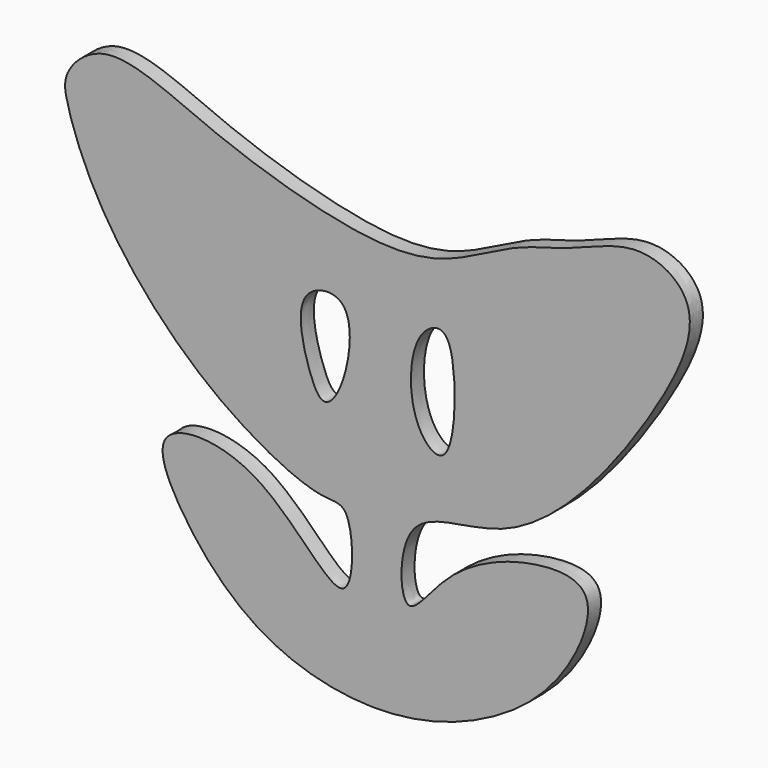
from build123d import *

# Parameters (mm, degrees)
F1_DEPTH = 2
F3_DEPTH = 25


with BuildPart() as f1:
    # F0 (on Front) → F1 (new body)
    with BuildSketch(Plane.XZ):
        with BuildLine():
            add(Edge.make_bspline(
                [(-75.8347990971, 56.2486425042), (-75.1836263652, 57.6802689805), (-70.9340790333, 61.7640658934), (-58.7880150697, 55.6323601286), (-43.4543911865, 50.6624350906), (-30.7629702937, 49.5047020163), (-21.2430871182, 55.7381469131), (-14.4280411182, 56.8600440589), (-5.9908935153, 61.2392779803), (2.5977107271, 56.1596013405), (-3.7766212938, 42.0301545009), (-19.9171824428, 21.4464982023), (-35.5090674399, 24.204165931), (-35.1659184419, 8.7502373537), (-29.3709449572, 18.4771355864), (-19.1906116712, 22.527164785), (-10.2486183797, 21.8239112152), (-14.7448810071, 9.9497124678), (-24.7301847276, 2.2972307162), (-37.8974817036, -1.1632111012), (-52.6991606842, 2.3225134129), (-61.8943580671, 12.4158839786), (-66.5312753548, 22.7161079835), (-51.5232135092, 22.7569790255), (-40.576550772, 5.5851938951), (-40.8518766389, 21.2862833862), (-45.3318688846, 20.0077827884), (-59.5970602772, 27.2946481454), (-71.9458419573, 41.6440588858), (-75.9609853522, 52.4043003525), (-76.3433099111, 55.1306633428), (-75.8347990971, 56.2486425042)],
                knots=[0, 0, 0, 0, 0.0253349266, 0.0628814506, 0.1064129014, 0.1436333956, 0.1780743263, 0.2061872931, 0.2378149533, 0.2655878625, 0.304558889, 0.3583719074, 0.3954019389, 0.4254899915, 0.4524182936, 0.4893046572, 0.5153680757, 0.5480343317, 0.586157669, 0.6246036867, 0.6649227249, 0.7046153879, 0.733595282, 0.7687775312, 0.8078125444, 0.8378755979, 0.8566485225, 0.8978413978, 0.9453852813, 0.9802155657, 1, 1, 1, 1], degree=3))
        make_face()
    extrude(amount=F1_DEPTH)

    # F2 (on face) → F3 (cut)
    with BuildSketch(Plane.XZ.offset(2)):
        with BuildLine():
            add(Edge.make_bspline(
                [(-42.2871634364, 42.2871671617), (-40.7233235578, 40.7460702061), (-41.6404243336, 33.64294769), (-44.5487515397, 29.883684324), (-46.6450188115, 34.0930294047), (-48.5043967712, 42.6275810256), (-43.3972597055, 43.3811193011), (-42.2871634364, 42.2871671617)],
                knots=[0, 0, 0, 0, 0.25425656, 0.4151017388, 0.5773983635, 0.8195152442, 1, 1, 1, 1], degree=3))
        make_face()
        with BuildLine():
            add(Edge.make_bspline(
                [(-32.8900180757, 41.4816960692), (-34.1259395093, 39.117633331), (-34.1810178637, 32.0726846499), (-28.7069781951, 27.6905511122), (-28.1052302328, 39.4105956249), (-29.6890897505, 44.3984102877), (-32.160134876, 42.8778120591), (-32.8900180757, 41.4816960692)],
                knots=[0, 0, 0, 0, 0.2565147826, 0.4164232009, 0.674236833, 0.8485131618, 1, 1, 1, 1], degree=3))
        make_face()
    extrude(amount=-F3_DEPTH, mode=Mode.SUBTRACT)


solid = f1.part
